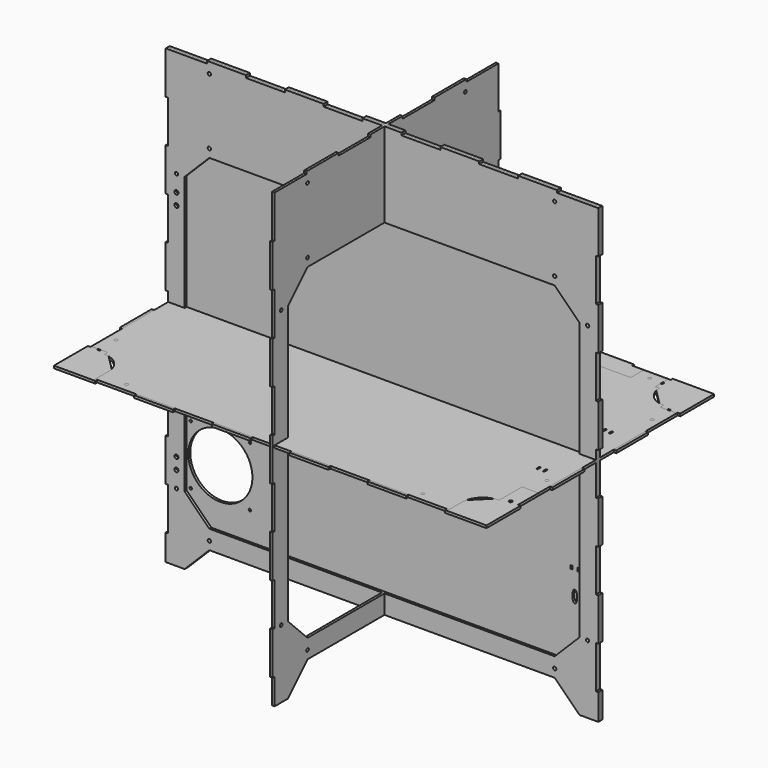
from build123d import *

# Parameters (mm, degrees)
F1_R     = 2
F2_DEPTH = 3
F3_R     = 2
F3_R_2   = 2.5
F4_DEPTH = 3
F3_R_3   = 1.5
F3_W     = 2
F3_H     = 4
F5_DEPTH = 3
F6_R     = 2
F6_R_2   = 2.5
F7_DEPTH = 3
F8_R     = 2
F8_W     = 2
F8_H     = 5
F9_DEPTH = 3


# Not quite as in the source:
# - a feature names something its author has since deleted; it is built from what else it names


with BuildPart() as f2:
    # F1 (on Top) → F2 (new body)
    with BuildSketch(Plane.XY):
        Polygon((212.7272727273, -173), (263, -173), (263, -121.4285714286), (260, -121.4285714286), (260, -72.8571428571), (263, -72.8571428571), (263, -24.2857142857), (260, -24.2857142857), (260, 24.2857142857), (263, 24.2857142857), (263, 72.8571428571), (260, 72.8571428571), (260, 121.4285714286), (263, 121.4285714286), (263, 173), (212.7272727273, 173), (212.7272727273, 170), (165.4545454545, 170), (165.4545454545, 173), (118.1818181818, 173), (118.1818181818, 170), (70.9090909091, 170), (70.9090909091, 173), (23.6363636364, 173), (23.6363636364, 170), (-23.6363636364, 170), (-23.6363636364, 173), (-70.9090909091, 173), (-70.9090909091, 170), (-118.1818181818, 170), (-118.1818181818, 173), (-165.4545454545, 173), (-165.4545454545, 170), (-212.7272727273, 170), (-212.7272727273, 173), (-263, 173), (-263, 121.4285714286), (-260, 121.4285714286), (-260, 72.8571428571), (-263, 72.8571428571), (-263, 24.2857142857), (-260, 24.2857142857), (-260, -24.2857142857), (-263, -24.2857142857), (-263, -72.8571428571), (-260, -72.8571428571), (-260, -121.4285714286), (-263, -121.4285714286), (-263, -173), (-212.7272727273, -173), (-212.7272727273, -170), (-165.4545454545, -170), (-165.4545454545, -173), (-118.1818181818, -173), (-118.1818181818, -170), (-70.9090909091, -170), (-70.9090909091, -173), (-23.6363636364, -173), (-23.6363636364, -170), (23.6363636364, -170), (23.6363636364, -173), (70.9090909091, -173), (70.9090909091, -170), (118.1818181818, -170), (118.1818181818, -173), (165.4545454545, -173), (165.4545454545, -170), (212.7272727273, -170), align=None)
        with Locations((-210, -160)):
            Circle(F1_R, mode=Mode.SUBTRACT)
        with Locations((-250, -120)):
            Circle(F1_R, mode=Mode.SUBTRACT)
        with Locations((210, -160)):
            Circle(F1_R, mode=Mode.SUBTRACT)
        with Locations((250, -120)):
            Circle(F1_R, mode=Mode.SUBTRACT)
        with Locations((-250, 120)):
            Circle(F1_R, mode=Mode.SUBTRACT)
        with Locations((-210, 160)):
            Circle(F1_R, mode=Mode.SUBTRACT)
        Polygon((240, -120), (210, -150), (-210, -150), (-240, -120), (-240, 120), (-210, 150), (210, 150), (240, 120), align=None, mode=Mode.SUBTRACT)
        with Locations((250, 120)):
            Circle(F1_R, mode=Mode.SUBTRACT)
        with Locations((210, 160)):
            Circle(F1_R, mode=Mode.SUBTRACT)
    extrude(amount=F2_DEPTH)


with BuildPart() as f4:
    # F3 (on Front) → F4 (new body)
    with BuildSketch(Plane.XZ):
        Polygon((240, -276.5), (263, -276.5), (263, -244.6818181818), (260, -244.6818181818), (260, -192.8636363636), (263, -192.8636363636), (263, -141.0454545455), (260, -141.0454545455), (260, -89.2272727273), (263, -89.2272727273), (263, -37.4090909091), (260, -37.4090909091), (260, 14.4090909091), (263, 14.4090909091), (263, 66.2272727273), (260, 66.2272727273), (260, 118.0454545455), (263, 118.0454545455), (263, 169.8636363636), (260, 169.8636363636), (260, 221.6818181818), (263, 221.6818181818), (263, 273.5), (260, 273.5), (212.7272727273, 273.5), (212.7272727273, 276.5), (165.4545454545, 276.5), (165.4545454545, 273.5), (118.1818181818, 273.5), (118.1818181818, 276.5), (70.9090909091, 276.5), (70.9090909091, 273.5), (23.6363636364, 273.5), (23.6363636364, 276.5), (-23.6363636364, 276.5), (-23.6363636364, 273.5), (-70.9090909091, 273.5), (-70.9090909091, 276.5), (-118.1818181818, 276.5), (-118.1818181818, 273.5), (-165.4545454545, 273.5), (-165.4545454545, 276.5), (-212.7272727273, 276.5), (-212.7272727273, 273.5), (-260, 273.5), (-263, 273.5), (-263, 221.6818181818), (-260, 221.6818181818), (-260, 169.8636363636), (-263, 169.8636363636), (-263, 118.0454545455), (-260, 118.0454545455), (-260, 66.2272727273), (-263, 66.2272727273), (-263, 14.4090909091), (-260, 14.4090909091), (-260, -37.4090909091), (-263, -37.4090909091), (-263, -89.2272727273), (-260, -89.2272727273), (-260, -141.0454545455), (-263, -141.0454545455), (-263, -192.8636363636), (-260, -192.8636363636), (-260, -244.6818181818), (-263, -244.6818181818), (-263, -276.5), (-240, -276.5), (-210, -246.5), (210, -246.5), align=None)
        with Locations((-210, -236.5)):
            Circle(F3_R, mode=Mode.SUBTRACT)
        with Locations((-250, -193.5)):
            Circle(F3_R, mode=Mode.SUBTRACT)
        with Locations((-250, -173.5)):
            Circle(F3_R_2, mode=Mode.SUBTRACT)
        with Locations((-250, -159.5)):
            Circle(F3_R_2, mode=Mode.SUBTRACT)
        with Locations((210, -236.5)):
            Circle(F3_R, mode=Mode.SUBTRACT)
        with Locations((250, -193.5)):
            Circle(F3_R, mode=Mode.SUBTRACT)
        Polygon((-210, 173.5), (210, 173.5), (240, 143.5), (240, -193.5), (210, -223.5), (-210, -223.5), (-240, -193.5), (-240, 143.5), align=None, mode=Mode.SUBTRACT)
        with Locations((-250, 98.5)):
            Circle(F3_R, mode=Mode.SUBTRACT)
        with Locations((-250, 109.5)):
            Circle(F3_R_2, mode=Mode.SUBTRACT)
        with Locations((-250, 123.5)):
            Circle(F3_R_2, mode=Mode.SUBTRACT)
        with Locations((-250, 143.5)):
            Circle(F3_R, mode=Mode.SUBTRACT)
        with Locations((-210, 183.5)):
            Circle(F3_R, mode=Mode.SUBTRACT)
        with Locations((-210, 263.5)):
            Circle(F3_R, mode=Mode.SUBTRACT)
        with Locations((-190, 263.5)):
            Circle(F3_R_2, mode=Mode.SUBTRACT)
        with Locations((-176, 263.5)):
            Circle(F3_R_2, mode=Mode.SUBTRACT)
        with Locations((250, 98.5)):
            Circle(F3_R, mode=Mode.SUBTRACT)
        with Locations((250, 143.5)):
            Circle(F3_R, mode=Mode.SUBTRACT)
        with Locations((210, 183.5)):
            Circle(F3_R, mode=Mode.SUBTRACT)
        with Locations((176, 263.5)):
            Circle(F3_R_2, mode=Mode.SUBTRACT)
        with Locations((190, 263.5)):
            Circle(F3_R_2, mode=Mode.SUBTRACT)
        with Locations((210, 263.5)):
            Circle(F3_R, mode=Mode.SUBTRACT)
        with Locations((-190, 263.5)):
            Circle(F3_R_2)
        with Locations((-176, 263.5)):
            Circle(F3_R_2)
        with Locations((176, 263.5)):
            Circle(F3_R_2)
        with Locations((190, 263.5)):
            Circle(F3_R_2)
        with Locations((-250, 98.5)):
            Circle(F3_R)
        with Locations((250, 98.5)):
            Circle(F3_R)
    extrude(amount=F4_DEPTH)


with BuildPart() as f5:
    # F3 (on Front) → F5 (new body)
    with BuildSketch(Plane.XZ):
        Polygon((240, -276.5), (263, -276.5), (263, -244.6818181818), (260, -244.6818181818), (260, -192.8636363636), (263, -192.8636363636), (263, -141.0454545455), (260, -141.0454545455), (260, -89.2272727273), (263, -89.2272727273), (263, -37.4090909091), (260, -37.4090909091), (260, 14.4090909091), (263, 14.4090909091), (263, 66.2272727273), (260, 66.2272727273), (260, 118.0454545455), (263, 118.0454545455), (263, 169.8636363636), (260, 169.8636363636), (260, 221.6818181818), (263, 221.6818181818), (263, 273.5), (260, 273.5), (212.7272727273, 273.5), (212.7272727273, 276.5), (165.4545454545, 276.5), (165.4545454545, 273.5), (118.1818181818, 273.5), (118.1818181818, 276.5), (70.9090909091, 276.5), (70.9090909091, 273.5), (23.6363636364, 273.5), (23.6363636364, 276.5), (-23.6363636364, 276.5), (-23.6363636364, 273.5), (-70.9090909091, 273.5), (-70.9090909091, 276.5), (-118.1818181818, 276.5), (-118.1818181818, 273.5), (-165.4545454545, 273.5), (-165.4545454545, 276.5), (-212.7272727273, 276.5), (-212.7272727273, 273.5), (-260, 273.5), (-263, 273.5), (-263, 221.6818181818), (-260, 221.6818181818), (-260, 169.8636363636), (-263, 169.8636363636), (-263, 118.0454545455), (-260, 118.0454545455), (-260, 66.2272727273), (-263, 66.2272727273), (-263, 14.4090909091), (-260, 14.4090909091), (-260, -37.4090909091), (-263, -37.4090909091), (-263, -89.2272727273), (-260, -89.2272727273), (-260, -141.0454545455), (-263, -141.0454545455), (-263, -192.8636363636), (-260, -192.8636363636), (-260, -244.6818181818), (-263, -244.6818181818), (-263, -276.5), (-240, -276.5), (-210, -246.5), (210, -246.5), align=None)
        with Locations((-210, -236.5)):
            Circle(F3_R, mode=Mode.SUBTRACT)
        with Locations((-250, -193.5)):
            Circle(F3_R, mode=Mode.SUBTRACT)
        with Locations((-250, -173.5)):
            Circle(F3_R_2, mode=Mode.SUBTRACT)
        with Locations((-250, -159.5)):
            Circle(F3_R_2, mode=Mode.SUBTRACT)
        with Locations((210, -236.5)):
            Circle(F3_R, mode=Mode.SUBTRACT)
        with Locations((250, -193.5)):
            Circle(F3_R, mode=Mode.SUBTRACT)
        Polygon((-210, 173.5), (210, 173.5), (240, 143.5), (240, -193.5), (210, -223.5), (-210, -223.5), (-240, -193.5), (-240, 143.5), align=None, mode=Mode.SUBTRACT)
        with Locations((-250, 98.5)):
            Circle(F3_R, mode=Mode.SUBTRACT)
        with Locations((-250, 109.5)):
            Circle(F3_R_2, mode=Mode.SUBTRACT)
        with Locations((-250, 123.5)):
            Circle(F3_R_2, mode=Mode.SUBTRACT)
        with Locations((-250, 143.5)):
            Circle(F3_R, mode=Mode.SUBTRACT)
        with Locations((-210, 183.5)):
            Circle(F3_R, mode=Mode.SUBTRACT)
        with Locations((-210, 263.5)):
            Circle(F3_R, mode=Mode.SUBTRACT)
        with Locations((-190, 263.5)):
            Circle(F3_R_2, mode=Mode.SUBTRACT)
        with Locations((-176, 263.5)):
            Circle(F3_R_2, mode=Mode.SUBTRACT)
        with Locations((250, 98.5)):
            Circle(F3_R, mode=Mode.SUBTRACT)
        with Locations((250, 143.5)):
            Circle(F3_R, mode=Mode.SUBTRACT)
        with Locations((210, 183.5)):
            Circle(F3_R, mode=Mode.SUBTRACT)
        with Locations((176, 263.5)):
            Circle(F3_R_2, mode=Mode.SUBTRACT)
        with Locations((190, 263.5)):
            Circle(F3_R_2, mode=Mode.SUBTRACT)
        with Locations((210, 263.5)):
            Circle(F3_R, mode=Mode.SUBTRACT)
        Polygon((240, 143.5), (210, 173.5), (-210, 173.5), (-240, 143.5), (-240, -193.5), (-210, -223.5), (210, -223.5), (240, -193.5), align=None)
        with Locations((-235, -189.5)):
            Circle(F3_R_3, mode=Mode.SUBTRACT)
        with BuildLine():
            ThreePointArc((-232.4998083752, -173.4690470184), (-209.3563379958, -115.9001826691), (-160, -153.5))
            ThreePointArc((-160, -153.5), (-187.3185248302, -190.7094495775), (-231.0022121979, -175.7903210933))
            ThreePointArc((-231.0022121979, -175.7903210933), (-232.1007416206, -174.8553171746), (-232.4998083752, -173.4690470184))
        make_face(mode=Mode.SUBTRACT)
        with Locations((-163, -189.5)):
            Circle(F3_R_3, mode=Mode.SUBTRACT)
        with Locations((-235, -117.5)):
            Circle(F3_R_3, mode=Mode.SUBTRACT)
        with Locations((-163, -117.5)):
            Circle(F3_R_3, mode=Mode.SUBTRACT)
        with BuildLine():
            add(Edge.make_bspline(
                [(232, -161), (237.1961524227, -161), (234.5980762114, -149.75), (232, -138.5), (229.4019237886, -149.75), (226.8038475773, -161), (232, -161)],
                knots=[0, 0, 0, 2.0943951024, 2.0943951024, 4.1887902048, 4.1887902048, 6.2831853072, 6.2831853072, 6.2831853072], degree=2, weights=[1, 0.5, 1, 0.5, 1, 0.5, 1]))
        make_face(mode=Mode.SUBTRACT)
        with Locations((228, -123.5)):
            Rectangle(F3_W, F3_H, mode=Mode.SUBTRACT)
        with Locations((236, -123.5)):
            Rectangle(F3_W, F3_H, mode=Mode.SUBTRACT)
        with BuildLine():
            Line((210, -20), (210, -15))
            ThreePointArc((210, -15), (220, -25), (210, -35))
            Line((210, -35), (210, -30))
            ThreePointArc((210, -30), (205, -25), (210, -20))
        make_face(mode=Mode.SUBTRACT)
        with Locations((-230, 109.5)):
            Circle(F3_R_2, mode=Mode.SUBTRACT)
        with Locations((-230, 123.5)):
            Circle(F3_R_2, mode=Mode.SUBTRACT)
        with Locations((-250, 123.5)):
            Circle(F3_R_2)
        with Locations((-250, -159.5)):
            Circle(F3_R_2)
        with Locations((-250, -173.5)):
            Circle(F3_R_2)
        with BuildLine():
            ThreePointArc((210, -35), (220, -25), (210, -15))
            Line((210, -15), (210, -20))
            ThreePointArc((210, -20), (205, -25), (210, -30))
            Line((210, -30), (210, -35))
        make_face()
        with Locations((-250, 109.5)):
            Circle(F3_R_2)
        with BuildLine():
            ThreePointArc((-231.0022121979, -175.7903210933), (-231.7715692807, -174.6429479231), (-232.4998083752, -173.4690470184))
            ThreePointArc((-232.4998083752, -173.4690470184), (-232.1007416206, -174.8553171746), (-231.0022121979, -175.7903210933))
        make_face()
        with Locations((-230, 123.5)):
            Circle(F3_R_2)
        with Locations((-230, 109.5)):
            Circle(F3_R_2)
    extrude(amount=-F5_DEPTH)


with BuildPart() as f7:
    # F6 (on Right) → F7 (new body)
    with BuildSketch(Plane.YZ):
        Polygon((-170, -276.5), (-150, -276.5), (-120, -246.5), (120, -246.5), (150, -276.5), (170, -276.5), (170, -244.6818181818), (173, -244.6818181818), (173, -192.8636363636), (170, -192.8636363636), (170, -141.0454545455), (173, -141.0454545455), (173, -89.2272727273), (170, -89.2272727273), (170, -37.4090909091), (173, -37.4090909091), (173, 14.4090909091), (170, 14.4090909091), (170, 66.2272727273), (173, 66.2272727273), (173, 118.0454545455), (170, 118.0454545455), (170, 169.8636363636), (173, 169.8636363636), (173, 221.6818181818), (170, 221.6818181818), (170, 273.5), (121.4285714286, 273.5), (121.4285714286, 276.5), (72.8571428571, 276.5), (72.8571428571, 273.5), (24.2857142857, 273.5), (24.2857142857, 276.5), (-24.2857142857, 276.5), (-24.2857142857, 273.5), (-72.8571428571, 273.5), (-72.8571428571, 276.5), (-121.4285714286, 276.5), (-121.4285714286, 273.5), (-170, 273.5), (-170, 221.6818181818), (-173, 221.6818181818), (-173, 169.8636363636), (-170, 169.8636363636), (-170, 118.0454545455), (-173, 118.0454545455), (-173, 66.2272727273), (-170, 66.2272727273), (-170, 14.4090909091), (-173, 14.4090909091), (-173, -37.4090909091), (-170, -37.4090909091), (-170, -89.2272727273), (-173, -89.2272727273), (-173, -141.0454545455), (-170, -141.0454545455), (-170, -192.8636363636), (-173, -192.8636363636), (-173, -244.6818181818), (-170, -244.6818181818), align=None)
        with Locations((-120, -236.5)):
            Circle(F6_R, mode=Mode.SUBTRACT)
        with Locations((-160, -193.5)):
            Circle(F6_R, mode=Mode.SUBTRACT)
        with Locations((120, -236.5)):
            Circle(F6_R, mode=Mode.SUBTRACT)
        with Locations((160, -193.5)):
            Circle(F6_R, mode=Mode.SUBTRACT)
        with Locations((160, -173.5)):
            Circle(F6_R_2, mode=Mode.SUBTRACT)
        with Locations((160, -159.5)):
            Circle(F6_R_2, mode=Mode.SUBTRACT)
        Polygon((-150, 143.5), (-120, 173.5), (120, 173.5), (150, 143.5), (150, -193.5), (120, -223.5), (-120, -223.5), (-150, -193.5), align=None, mode=Mode.SUBTRACT)
        with Locations((-160, 143.5)):
            Circle(F6_R, mode=Mode.SUBTRACT)
        with Locations((-120, 183.5)):
            Circle(F6_R, mode=Mode.SUBTRACT)
        with Locations((-120, 263.5)):
            Circle(F6_R, mode=Mode.SUBTRACT)
        with Locations((160, 109.5)):
            Circle(F6_R_2, mode=Mode.SUBTRACT)
        with Locations((160, 123.5)):
            Circle(F6_R_2, mode=Mode.SUBTRACT)
        with Locations((120, 183.5)):
            Circle(F6_R, mode=Mode.SUBTRACT)
        with Locations((160, 143.5)):
            Circle(F6_R, mode=Mode.SUBTRACT)
        with Locations((120, 263.5)):
            Circle(F6_R, mode=Mode.SUBTRACT)
    extrude(amount=F7_DEPTH)


with BuildPart() as f9:
    # F8 (on Top) → F9 (new body)
    with BuildSketch(Plane.XY):
        with BuildLine():
            Line((215, -170), (215, -150))
            ThreePointArc((215, -150), (222.3223304703, -132.3223304703), (240, -125))
            Line((240, -125), (240, -90))
            Line((240, -90), (260, -90))
            Line((260, -90), (260, 120))
            Line((260, 120), (240, 120))
            Line((240, 120), (240, 125))
            ThreePointArc((240, 125), (222.3223304703, 132.3223304703), (215, 150))
            Line((215, 150), (210, 150))
            Line((210, 150), (210, 170))
            Line((210, 170), (180, 170))
            Line((180, 170), (180, 150))
            Line((180, 150), (37.5, 150))
            Line((37.5, 150), (37.5, 146.8))
            Line((37.5, 146.8), (24.5, 146.8))
            Line((24.5, 146.8), (24.5, 107))
            Line((24.5, 107), (-24.5, 107))
            Line((-24.5, 107), (-24.5, 146.8))
            Line((-24.5, 146.8), (-37.5, 146.8))
            Line((-37.5, 146.8), (-37.5, 150))
            Line((-37.5, 150), (-180, 150))
            Line((-180, 150), (-180, 170))
            Line((-180, 170), (-210, 170))
            Line((-210, 170), (-210, 150))
            Line((-210, 150), (-215, 150))
            ThreePointArc((-215, 150), (-222.3223304703, 132.3223304703), (-240, 125))
            Line((-240, 125), (-240, 90))
            Line((-240, 90), (-260, 90))
            Line((-260, 90), (-260, -120))
            Line((-260, -120), (-240, -120))
            Line((-240, -120), (-240, -125))
            ThreePointArc((-240, -125), (-222.3223304703, -132.3223304703), (-215, -150))
            Line((-215, -150), (-215, -170))
            Line((-215, -170), (215, -170))
        make_face()
        with Locations((-185, -160)):
            Circle(F8_R, mode=Mode.SUBTRACT)
        with Locations((-250, -95)):
            Circle(F8_R, mode=Mode.SUBTRACT)
        with Locations((175, -160)):
            Circle(F8_R, mode=Mode.SUBTRACT)
        with Locations((250, -65)):
            Circle(F8_R, mode=Mode.SUBTRACT)
        with Locations((228, -50)):
            Rectangle(F8_W, F8_H, mode=Mode.SUBTRACT)
        with Locations((236, -50)):
            Rectangle(F8_W, F8_H, mode=Mode.SUBTRACT)
        with Locations((-250, 65)):
            Circle(F8_R, mode=Mode.SUBTRACT)
        with Locations((-195, 160)):
            Circle(F8_R, mode=Mode.SUBTRACT)
        with Locations((228, 50)):
            Rectangle(F8_W, F8_H, mode=Mode.SUBTRACT)
        with Locations((236, 50)):
            Rectangle(F8_W, F8_H, mode=Mode.SUBTRACT)
        with Locations((250, 95)):
            Circle(F8_R, mode=Mode.SUBTRACT)
        with Locations((195, 160)):
            Circle(F8_R, mode=Mode.SUBTRACT)
    extrude(amount=F9_DEPTH)


solid = Compound([f2.part, f4.part, f5.part, f7.part, f9.part])
